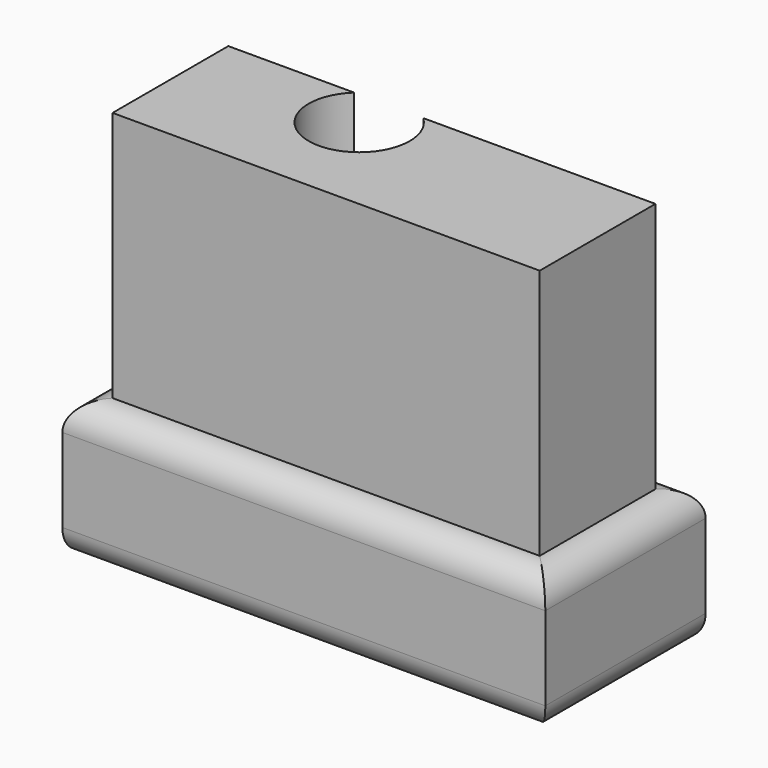
from build123d import *

# Parameters (mm, degrees)
F0_W        = 87.937258184
F0_H        = 36.5022588521
F0_R        = 9.2048285636
F1_DEPTH    = 25.4
F2_T1_DEPTH = 113.337258184
F2_T3_DEPTH = 61.9022588521
F3_DEPTH    = 45.72


# Not quite as in the source:
# - a fillet or chamfer that OpenCascade refuses, or shapes differently, is made with other operations: its cross-section is extruded or revolved along the edge and cut away or added


with BuildPart() as f1:
    # F0 (on Top) → F1 (new body)
    with BuildSketch(Plane.XY):
        with Locations((-1.4748387039, -2.3044357076)):
            Rectangle(F0_W, F0_H)
        with Locations((-11.1534688622, 4.1479840875)):
            Circle(F0_R, mode=Mode.SUBTRACT)
    extrude(amount=F1_DEPTH)

    # F2: fillet of radius 5.08 on 6 edges, made by hand

    # F2_s2 → F2_t1 (cut)
    with BuildSketch(Plane.YZ.offset(-58.1434677958)):
        with BuildLine():
            ThreePointArc((-20.5555651337, 20.32), (-19.0676675821, 23.9121024484), (-15.4755651337, 25.4))
            Line((-15.4755651337, 25.4), (-20.5555651337, 25.4))
            Line((-20.5555651337, 25.4), (-20.5555651337, 20.32))
        make_face()
        with BuildLine():
            ThreePointArc((15.9466937184, 20.32), (14.4587961669, 23.9121024484), (10.8666937184, 25.4))
            Line((10.8666937184, 25.4), (15.9466937184, 25.4))
            Line((15.9466937184, 25.4), (15.9466937184, 20.32))
        make_face()
        with BuildLine():
            ThreePointArc((-20.5555651337, 5.08), (-19.0676675821, 1.4878975516), (-15.4755651337, 0))
            Line((-15.4755651337, 0), (-20.5555651337, 0))
            Line((-20.5555651337, 0), (-20.5555651337, 5.08))
        make_face()
    extrude(amount=F2_T1_DEPTH, mode=Mode.SUBTRACT)

    # F2_s4 → F2_t3 (cut)
    with BuildSketch(Plane.XZ.offset(-28.6466937184)):
        with BuildLine():
            ThreePointArc((-45.4434677958, 20.32), (-43.9555702443, 23.9121024484), (-40.3634677958, 25.4))
            Line((-40.3634677958, 25.4), (-45.4434677958, 25.4))
            Line((-45.4434677958, 25.4), (-45.4434677958, 20.32))
        make_face()
        with BuildLine():
            ThreePointArc((42.4937903881, 20.32), (41.0058928365, 23.9121024484), (37.4137903881, 25.4))
            Line((37.4137903881, 25.4), (42.4937903881, 25.4))
            Line((42.4937903881, 25.4), (42.4937903881, 20.32))
        make_face()
        with BuildLine():
            ThreePointArc((42.4937903881, 5.08), (41.0058928365, 1.4878975516), (37.4137903881, 0))
            Line((37.4137903881, 0), (42.4937903881, 0))
            Line((42.4937903881, 0), (42.4937903881, 5.08))
        make_face()
    extrude(amount=F2_T3_DEPTH, mode=Mode.SUBTRACT)

    # F3 (add): a face of the model
    f3_faces = [f1.faces().sort_by_distance(p)[0] for p in [
        (-0.1621567776, -3.0875160288, 25.4),
    ]]
    extrude(f3_faces, amount=F3_DEPTH)


solid = f1.part
